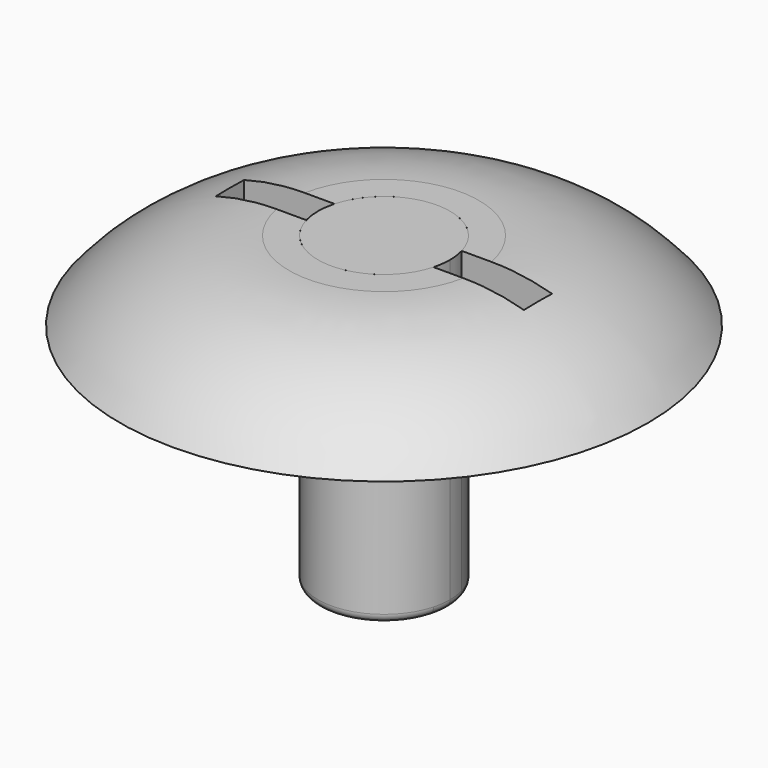
from build123d import *

# Parameters (mm, degrees)
F1_DEPTH      = 10
F1_DEPTH_BACK = 25
F2_START      = 1
F0_R          = 30
F2_DEPTH      = 9
F4_R          = 1
F5_START      = 1
F5_DEPTH      = 2


# Not quite as in the source:
# - a fillet or chamfer that OpenCascade refuses, or shapes differently, is made with other operations: its cross-section is extruded or revolved along the edge and cut away or added


with BuildPart() as f1:
    # F0 (on Top) → F1 (new body, two sides)
    with BuildSketch(Plane.XY) as f1_sk:
        with BuildLine():
            ThreePointArc((7.2284161474, -2), (7.4317938987, -1.0091776094), (7.5, 0))
            ThreePointArc((7.5, 0), (7.4317938987, 1.0091776094), (7.2284161474, 2))
            Line((7.2284161474, 2), (-7.2284161474, 2))
            ThreePointArc((-7.2284161474, 2), (-7.5, 0), (-7.2284161474, -2))
            Line((-7.2284161474, -2), (7.2284161474, -2))
        make_face()
        with BuildLine():
            ThreePointArc((-7.2284161474, -2), (0, -7.5), (7.2284161474, -2))
            Line((7.2284161474, -2), (-7.2284161474, -2))
        make_face()
        with BuildLine():
            Line((-7.2284161474, 2), (7.2284161474, 2))
            ThreePointArc((7.2284161474, 2), (0, 7.5), (-7.2284161474, 2))
        make_face()
    extrude(amount=F1_DEPTH)
    extrude(f1_sk.sketch, amount=-F1_DEPTH_BACK)

    # F4
    f4_edges = [f1.edges().sort_by_distance(p)[0] for p in [
        (-7.228416, -2, -25),
    ]]
    fillet(f4_edges, radius=F4_R)


with BuildPart() as f2:
    # F0 (on Top) → F2 (new body)
    with BuildSketch(Plane.XY.offset(F2_START)):
        Circle(F0_R)
        with BuildLine():
            ThreePointArc((-7.2284161474, 2), (0, 7.5), (7.2284161474, 2))
            Line((7.2284161474, 2), (17.5, 2))
            Line((17.5, 2), (17.5, -2))
            Line((17.5, -2), (7.2284161474, -2))
            ThreePointArc((7.2284161474, -2), (0, -7.5), (-7.2284161474, -2))
            Line((-7.2284161474, -2), (-17.5, -2))
            Line((-17.5, -2), (-17.5, 2))
            Line((-17.5, 2), (-7.2284161474, 2))
        make_face(mode=Mode.SUBTRACT)
    extrude(amount=F2_DEPTH)

    # F3: fillet of radius 25 on 1 edges, made by hand

    # F3_s1 → F3_t2 (revolve, cut)
    with BuildSketch(Plane.XZ):
        with BuildLine():
            ThreePointArc((30, 1), (21.3972290055, 7.6384628453), (10.7906272877, 10))
            Line((10.7906272877, 10), (30, 10))
            Line((30, 10), (30, 1))
        make_face()
    revolve(axis=Axis((0, 0, 10), (0, 0, 1)), mode=Mode.SUBTRACT)


with BuildPart() as f5:
    # F0 (on Top) → F5 (new body)
    with BuildSketch(Plane.XY.offset(F5_START)):
        with BuildLine():
            ThreePointArc((-7.2284161474, -2), (-7.5, 0), (-7.2284161474, 2))
            Line((-7.2284161474, 2), (-17.5, 2))
            Line((-17.5, 2), (-17.5, -2))
            Line((-17.5, -2), (-7.2284161474, -2))
        make_face()
    extrude(amount=F5_DEPTH)


with BuildPart() as f5b:
    # F0 (on Top) → F5, piece 2 (new body)
    with BuildSketch(Plane.XY.offset(F5_START)):
        with BuildLine():
            ThreePointArc((7.2284161474, 2), (7.4317938987, 1.0091776094), (7.5, 0))
            ThreePointArc((7.5, 0), (7.4317938987, -1.0091776094), (7.2284161474, -2))
            Line((7.2284161474, -2), (17.5, -2))
            Line((17.5, -2), (17.5, 2))
            Line((17.5, 2), (7.2284161474, 2))
        make_face()
    extrude(amount=F5_DEPTH)


solid = Compound([f1.part, f2.part, f5.part, f5b.part])
